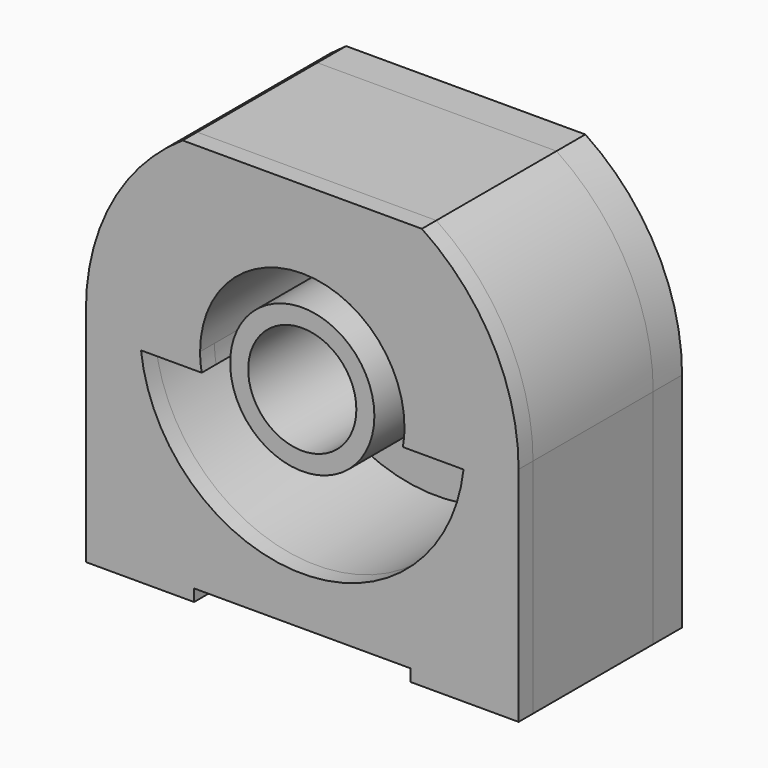
from build123d import *

# Parameters (mm, degrees)
F1_DEPTH = 28
F0_R     = 9
F2_DEPTH = 6
F3_DEPTH = 25


# Not quite as in the source:
# - a feature names something its author has since deleted; it is built from what else it names


with BuildPart() as f1:
    # F0 (on Front) → F1 (new body)
    with BuildSketch(Plane.XZ):
        with BuildLine():
            Line((0, 37), (0, 34))
            Line((0, 34), (9.16718427, 34))
            Line((9.16718427, 34), (9.6703589086, 34))
            Line((9.6703589086, 34), (16.2262800667, 34))
            Line((16.2262800667, 34), (19.2667994693, 34))
            ThreePointArc((19.2667994693, 34), (19.0668312324, 35.494079853), (19, 37))
            Line((19, 37), (9.5, 37))
            ThreePointArc((9.5, 37), (36, 63.5), (62.5, 37))
            Line((62.5, 37), (53, 37))
            ThreePointArc((53, 37), (52.9331687676, 35.494079853), (52.7332005307, 34))
            Line((52.7332005307, 34), (62.83281573, 34))
            Line((62.83281573, 34), (72, 34))
            Line((72, 34), (72, 37))
            ThreePointArc((72, 37), (67.7205844423, 54.0236459856), (55.8997487421, 67))
            Line((55.8997487421, 67), (16.1002512579, 67))
            ThreePointArc((16.1002512579, 67), (4.2794155577, 54.0236459856), (0, 37))
        make_face()
        with BuildLine():
            ThreePointArc((19, 37), (36, 54), (53, 37))
            Line((53, 37), (62.5, 37))
            ThreePointArc((62.5, 37), (36, 63.5), (9.5, 37))
            Line((9.5, 37), (19, 37))
        make_face()
        with BuildLine():
            Line((0, 34), (0, 0))
            Line((0, 0), (18, 0))
            Line((18, 0), (18, 2))
            Line((18, 2), (54, 2))
            Line((54, 2), (54, 0))
            Line((54, 0), (72, 0))
            Line((72, 0), (72, 34))
            Line((72, 34), (62.83281573, 34))
            ThreePointArc((62.83281573, 34), (36, 10), (9.16718427, 34))
            Line((9.16718427, 34), (0, 34))
        make_face()
    extrude(amount=F1_DEPTH)


with BuildPart() as f1b:
    # F0 (on Front) → F1, piece 2 (new body)
    with BuildSketch(Plane.XZ):
        with BuildLine():
            ThreePointArc((24, 37), (36, 25), (48, 37))
            ThreePointArc((48, 37), (36, 49), (24, 37))
        make_face()
        with Locations((36, 37)):
            Circle(F0_R, mode=Mode.SUBTRACT)
    extrude(amount=F1_DEPTH)


with BuildPart() as f2:
    # F0 (on Front) → F2 (new body)
    with BuildSketch(Plane.XZ):
        with BuildLine():
            ThreePointArc((19, 37), (36, 54), (53, 37))
            Line((53, 37), (62.5, 37))
            ThreePointArc((62.5, 37), (36, 63.5), (9.5, 37))
            Line((9.5, 37), (19, 37))
        make_face()
        with BuildLine():
            Line((0, 37), (0, 34))
            Line((0, 34), (9.16718427, 34))
            Line((9.16718427, 34), (9.6703589086, 34))
            Line((9.6703589086, 34), (16.2262800667, 34))
            Line((16.2262800667, 34), (19.2667994693, 34))
            ThreePointArc((19.2667994693, 34), (19.0668312324, 35.494079853), (19, 37))
            Line((19, 37), (9.5, 37))
            ThreePointArc((9.5, 37), (36, 63.5), (62.5, 37))
            Line((62.5, 37), (53, 37))
            ThreePointArc((53, 37), (52.9331687676, 35.494079853), (52.7332005307, 34))
            Line((52.7332005307, 34), (62.83281573, 34))
            Line((62.83281573, 34), (72, 34))
            Line((72, 34), (72, 37))
            ThreePointArc((72, 37), (67.7205844423, 54.0236459856), (55.8997487421, 67))
            Line((55.8997487421, 67), (16.1002512579, 67))
            ThreePointArc((16.1002512579, 67), (4.2794155577, 54.0236459856), (0, 37))
        make_face()
        with BuildLine():
            Line((0, 34), (0, 0))
            Line((0, 0), (18, 0))
            Line((18, 0), (18, 2))
            Line((18, 2), (54, 2))
            Line((54, 2), (54, 0))
            Line((54, 0), (72, 0))
            Line((72, 0), (72, 34))
            Line((72, 34), (62.83281573, 34))
            ThreePointArc((62.83281573, 34), (36, 10), (9.16718427, 34))
            Line((9.16718427, 34), (0, 34))
        make_face()
        with BuildLine():
            Line((9.6703589086, 34), (9.16718427, 34))
            ThreePointArc((9.16718427, 34), (36, 10), (62.83281573, 34))
            Line((62.83281573, 34), (52.7332005307, 34))
            ThreePointArc((52.7332005307, 34), (36, 20), (19.2667994693, 34))
            Line((19.2667994693, 34), (16.2262800667, 34))
            Line((16.2262800667, 34), (9.6703589086, 34))
        make_face()
    extrude(amount=-F2_DEPTH)


with BuildPart() as f3:
    # F0 (on Front) → F3 (new body)
    with BuildSketch(Plane.XZ):
        with BuildLine():
            Line((0, 34), (0, 0))
            Line((0, 0), (18, 0))
            Line((18, 0), (18, 2))
            Line((18, 2), (54, 2))
            Line((54, 2), (54, 0))
            Line((54, 0), (72, 0))
            Line((72, 0), (72, 34))
            Line((72, 34), (62.83281573, 34))
            ThreePointArc((62.83281573, 34), (36, 10), (9.16718427, 34))
            Line((9.16718427, 34), (0, 34))
        make_face()
        with BuildLine():
            Line((0, 37), (0, 34))
            Line((0, 34), (9.16718427, 34))
            Line((9.16718427, 34), (9.6703589086, 34))
            Line((9.6703589086, 34), (16.2262800667, 34))
            Line((16.2262800667, 34), (19.2667994693, 34))
            ThreePointArc((19.2667994693, 34), (19.0668312324, 35.494079853), (19, 37))
            Line((19, 37), (9.5, 37))
            ThreePointArc((9.5, 37), (36, 63.5), (62.5, 37))
            Line((62.5, 37), (53, 37))
            ThreePointArc((53, 37), (52.9331687676, 35.494079853), (52.7332005307, 34))
            Line((52.7332005307, 34), (62.83281573, 34))
            Line((62.83281573, 34), (72, 34))
            Line((72, 34), (72, 37))
            ThreePointArc((72, 37), (67.7205844423, 54.0236459856), (55.8997487421, 67))
            Line((55.8997487421, 67), (16.1002512579, 67))
            ThreePointArc((16.1002512579, 67), (4.2794155577, 54.0236459856), (0, 37))
        make_face()
    extrude(amount=F3_DEPTH)


solid = Compound([f1.part, f1b.part, f2.part, f3.part])
